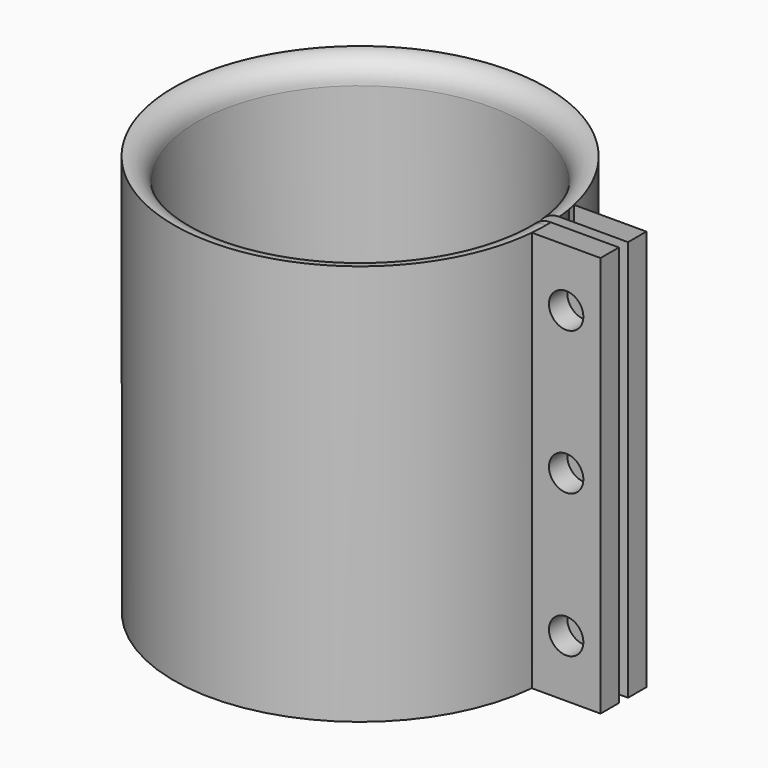
from build123d import *

# Parameters (mm, degrees)
F1_DEPTH = 35
F0_R     = 12.75
F2_DEPTH = 3
F0_R_2   = 11
F3_DEPTH = 2
F4_R     = 1.5
F5_DEPTH = 25
F6_R     = 1.99999


# Not quite as in the source:
# - a fillet or chamfer is up to 0.001 mm smaller than in the source, because OpenCascade refuses the exact size


with BuildPart() as f1:
    # F0 (on Top) → F1 (new body)
    with BuildSketch(Plane.XY):
        with BuildLine():
            ThreePointArc((14.2412253686, 0.5), (14.2478061733, 0.2500384941), (14.25, 0))
            ThreePointArc((14.25, 0), (-14.2301944166, -0.7510438499), (14.1708327208, 1.5))
            Line((14.1708327208, 1.5), (16.1806211253, 1.5))
            ThreePointArc((16.1806211253, 1.5), (16.055782786, 2.5048630957), (15.8686010726, 3.5))
            ThreePointArc((15.8686010726, 3.5), (-16.2184512476, -1.0120964027), (16.1806211253, -1.5))
            ThreePointArc((16.1806211253, -1.5), (16.2326460148, -0.7508018094), (16.25, 0))
            ThreePointArc((16.25, 0), (16.2480763538, 0.2500295981), (16.2423058708, 0.5))
            Line((16.2423058708, 0.5), (16.1806211253, 0.5))
            Line((16.1806211253, 0.5), (14.2412253686, 0.5))
        make_face()
        with BuildLine():
            ThreePointArc((15.8686010726, 3.5), (16.055782786, 2.5048630957), (16.1806211253, 1.5))
            Line((16.1806211253, 1.5), (22.1806211253, 1.5))
            Line((22.1806211253, 1.5), (22.1806211253, 3.5))
            Line((22.1806211253, 3.5), (15.8686010726, 3.5))
        make_face()
        with BuildLine():
            Line((22.1806211253, 0.5), (16.2423058708, 0.5))
            ThreePointArc((16.2423058708, 0.5), (16.2480763538, 0.2500295981), (16.25, 0))
            ThreePointArc((16.25, 0), (16.2326460148, -0.7508018094), (16.1806211253, -1.5))
            Line((16.1806211253, -1.5), (22.1806211253, -1.5))
            Line((22.1806211253, -1.5), (22.1806211253, 0.5))
        make_face()
    extrude(amount=F1_DEPTH)

    # F0 (on Top) → F2 (join)
    with BuildSketch(Plane.XY):
        with BuildLine():
            ThreePointArc((14.1708327208, 1.5), (-14.2301944166, -0.7510438499), (14.25, 0))
            ThreePointArc((14.25, 0), (14.2478061733, 0.2500384941), (14.2412253686, 0.5))
            ThreePointArc((14.2412253686, 0.5), (14.2148254023, 1.0006191989), (14.1708327208, 1.5))
        make_face()
        Circle(F0_R, mode=Mode.SUBTRACT)
    extrude(amount=F2_DEPTH)

    # F0 (on Top) → F3 (join)
    with BuildSketch(Plane.XY):
        Circle(F0_R)
        Circle(F0_R_2, mode=Mode.SUBTRACT)
    extrude(amount=F3_DEPTH)

    # F4 (on face) → F5 (cut)
    with BuildSketch(Plane.XZ.offset(1.5)):
        with Locations((19.1806211253, 30)):
            Circle(F4_R)
        with Locations((19.1806211253, 5)):
            Circle(F4_R)
        with Locations((19.1806211253, 17.5)):
            Circle(F4_R)
    extrude(amount=-F5_DEPTH, mode=Mode.SUBTRACT)

    # F6 (radius 2 in the source; OpenCascade refuses exactly that, so slightly less here)
    f6_edges = [f1.edges().sort_by_distance(p)[0] for p in [
        (-14.214825, -1.000619, 35),
    ]]
    fillet(f6_edges, radius=F6_R)


solid = f1.part
